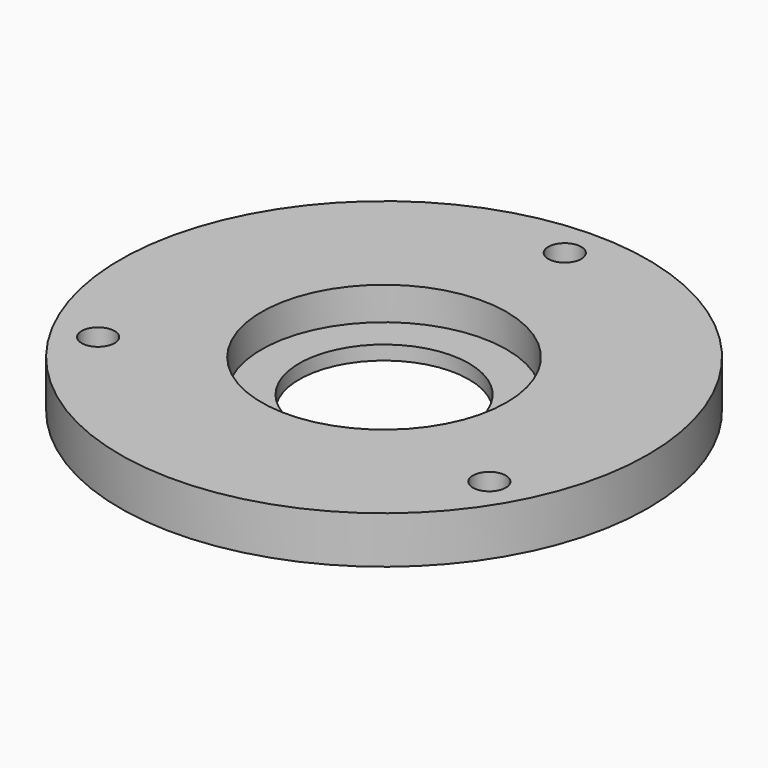
from build123d import *

# Parameters (mm, degrees)
F0_R     = 28
F0_R_2   = 1.75
F1_DEPTH = 5
F2_R     = 13
F3_DEPTH = 3.5
F4_R     = 9
F5_DEPTH = 1.501


# Not quite as in the source:
# - a feature names something its author has since deleted; it is built from what else it names


with BuildPart() as f1:
    # F0 (on Top) → F1 (new body)
    with BuildSketch(Plane.XY):
        Circle(F0_R)
        with Locations((-20.75, -11.9800180857)):
            Circle(F0_R_2, mode=Mode.SUBTRACT)
        with Locations((20.75, -11.9800180857)):
            Circle(F0_R_2, mode=Mode.SUBTRACT)
        with Locations((0, 23.9600361714)):
            Circle(F0_R_2, mode=Mode.SUBTRACT)
    extrude(amount=F1_DEPTH)

    # F2 (on face) → F3 (cut)
    with BuildSketch(Plane.XY.offset(5)):
        Circle(F2_R)
    extrude(amount=-F3_DEPTH, mode=Mode.SUBTRACT)

    # F4 (on face) → F5 (cut, through all)
    with BuildSketch(Plane.XY.offset(1.5)):
        Circle(F4_R)
    extrude(amount=-F5_DEPTH, mode=Mode.SUBTRACT)


solid = f1.part
